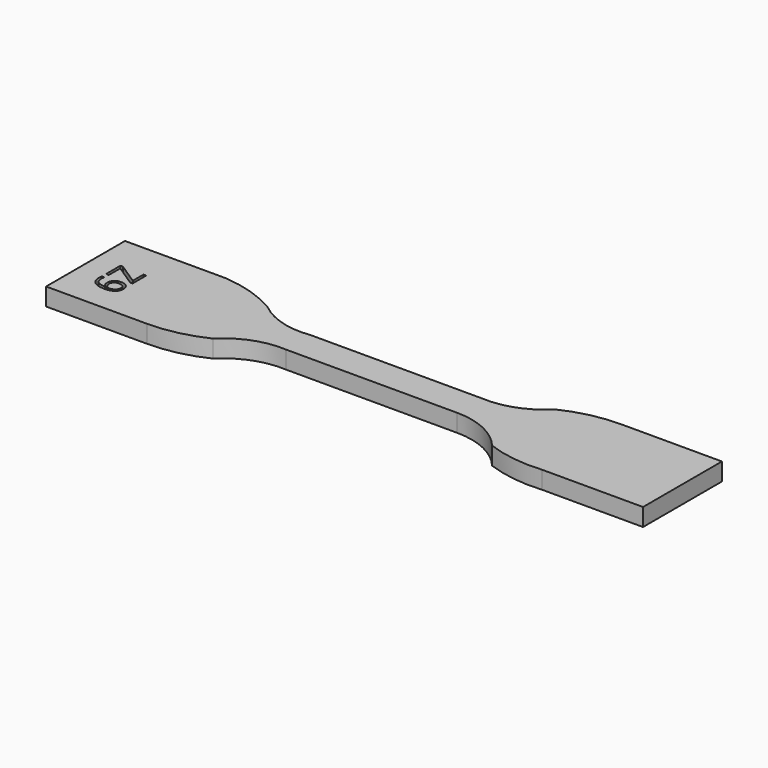
from build123d import *

# Parameters (mm, degrees)
F1_DEPTH     = 3.4
F2_TEXT_SIZE = 7.0564552314
F3_DEPTH     = 1


# Not quite as in the source:
# - Text() gives the source's letters only with a copy of the font that has no kerning and outlines rounded to 1/6400 em; it was checked with that copy


with BuildPart() as f1:
    # F0 (on Top) → F1 (new body)
    with BuildSketch(Plane.XY):
        with BuildLine():
            Line((-14.4320548165, 19.7811394548), (-33.8720548165, 19.7811394548))
            Line((-33.8720548165, 19.7811394548), (-33.8720548165, 0.7811394548))
            Line((-33.8720548165, 0.7811394548), (-14.4320548165, 0.7811394548))
            ThreePointArc((-14.4320548165, 0.7811394548), (-8.9053122052, 1.3996892086), (-3.6520548165, 3.2247301661))
            ThreePointArc((-3.6520548165, 3.2247301661), (1.3014698263, 6.4128780055), (7.1279451835, 7.2811394548))
            Line((7.1279451835, 7.2811394548), (40.1279451835, 7.2811394548))
            ThreePointArc((40.1279451835, 7.2811394548), (46.0837574042, 5.9511158081), (50.9079451835, 2.2137538538))
            ThreePointArc((50.9079451835, 2.2137538538), (56.2191047011, 0.9041953221), (61.6879451835, 0.7811394548))
            Line((61.6879451835, 0.7811394548), (81.1279451835, 0.7811394548))
            Line((81.1279451835, 0.7811394548), (81.1279451835, 19.7811394548))
            Line((81.1279451835, 19.7811394548), (61.6879451835, 19.7811394548))
            ThreePointArc((61.6879451835, 19.7811394548), (56.1612025723, 19.162589701), (50.9079451835, 17.3375487435))
            ThreePointArc((50.9079451835, 17.3375487435), (45.9544205407, 14.1494009041), (40.1279451835, 13.2811394548))
            Line((40.1279451835, 13.2811394548), (7.1279451835, 13.2811394548))
            ThreePointArc((7.1279451835, 13.2811394548), (1.4167452884, 13.6925537245), (-3.6520548165, 16.3560723447))
            ThreePointArc((-3.6520548165, 16.3560723447), (-8.8458057958, 18.686276846), (-14.4320548165, 19.7811394548))
        make_face()
    extrude(amount=F1_DEPTH)

    # F2 (on face) → F3 (cut)
    with BuildSketch(Plane.XY.offset(3.4)):
        with Locations(Location((-29.3720550835, 13.353464842), (0, 0, -90))):
            Text('Z9', F2_TEXT_SIZE, font='Open Sans', text_align=(TextAlign.LEFT, TextAlign.BOTTOM))
    extrude(amount=-F3_DEPTH, mode=Mode.SUBTRACT)


solid = f1.part
